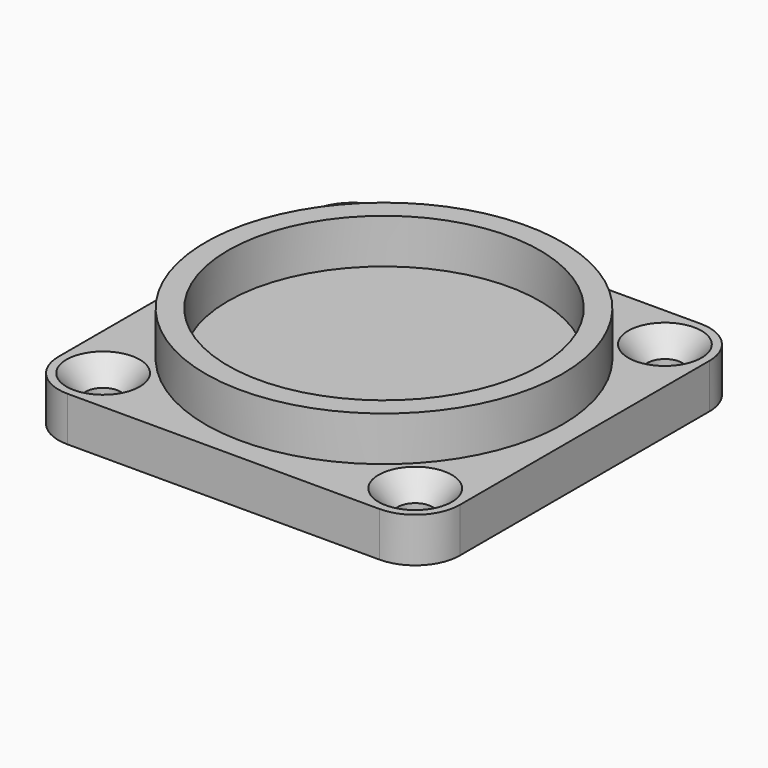
from build123d import *

# Parameters (mm, degrees)
F0_W           = 57.15
F0_H           = 57.15
F1_DEPTH       = 6.35
F3_D           = 4.9784
F3_CSINK_D     = 10.4394
F3_CSINK_ANGLE = 82
F4_R           = 25.4
F4_R_2         = 22.225
F5_DEPTH       = 6.35
F6_R           = 6.35


# Not quite as in the source:
# - a feature names something its author has since deleted; it is built from what else it names


with BuildPart() as f1:
    # F0 (on Top) → F1 (new body)
    with BuildSketch(Plane.XY):
        Rectangle(F0_W, F0_H)
    extrude(amount=F1_DEPTH)

    # F3 (through all)
    with Locations(Plane.XY.offset(6.35)):
        with Locations((-22.225, 22.225), (22.225, 22.225), (22.225, -22.225), (-22.225, -22.225)):
            CounterSinkHole(F3_D / 2, F3_CSINK_D / 2, counter_sink_angle=F3_CSINK_ANGLE)

    # F4 (on face) → F5 (join)
    with BuildSketch(Plane.XY.offset(6.35)):
        Circle(F4_R)
        Circle(F4_R_2, mode=Mode.SUBTRACT)
    extrude(amount=F5_DEPTH)

    # F6
    f6_edges = [f1.edges().sort_by_distance(p)[0] for p in [
        (28.575, 28.575, 3.175),
        (-28.575, 28.575, 3.175),
        (28.575, -28.575, 3.175),
        (-28.575, -28.575, 3.175),
    ]]
    fillet(f6_edges, radius=F6_R)


solid = f1.part
